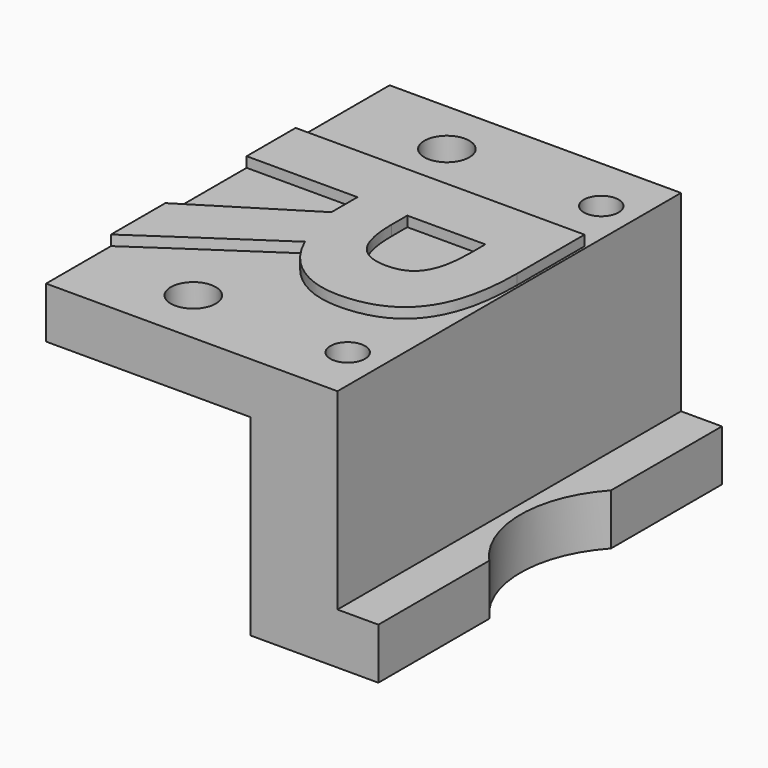
from build123d import *

# Parameters (mm, degrees)
F1_DEPTH     = 42
F2_R         = 1.7
F2_R_2       = 11
F3_DEPTH     = 23.801
F4_W         = 42
F4_H         = 5
F5_DEPTH     = 20
F6_R         = 2.2
F7_DEPTH     = 25
F8_TEXT_SIZE = 39.5833333333
F9_DEPTH     = 1


# Not quite as in the source:
# - Text() gives the source's letters only with a copy of the font that has no kerning and outlines rounded to 1/6400 em; it was checked with that copy


with BuildPart() as f1:
    # F0 (on Front) → F1 (new body)
    with BuildSketch(Plane.XZ):
        Polygon((8.5, 5), (8.5, 23.8), (0, 23.8), (0, 0), (12.5, 0), (12.5, 5), align=None)
    extrude(amount=-F1_DEPTH)

    # F2 (on face) → F3 (cut, through all)
    with BuildSketch(Plane(origin=(0, 0, 0), x_dir=(1, 0, 0), z_dir=(0, 0, -1))):
        with Locations((5.1, -5.5)):
            Circle(F2_R)
        with Locations((5.1, -36.5)):
            Circle(F2_R)
        with Locations((20.6, -21)):
            Circle(F2_R_2)
    extrude(amount=-F3_DEPTH, mode=Mode.SUBTRACT)

    # F4 (on face) → F5 (join)
    with BuildSketch(Plane(origin=(0, 0, 0), x_dir=(0, -1, 0), z_dir=(-1, 0, 0))):
        with Locations((-21, 21.3)):
            Rectangle(F4_W, F4_H)
    extrude(amount=F5_DEPTH)

    # F6 (on face) → F7 (cut)
    with BuildSketch(Plane.XY.offset(23.8)):
        with Locations((-10, 36.5)):
            Circle(F6_R)
        with Locations((-10, 5.5)):
            Circle(F6_R)
    extrude(amount=-F7_DEPTH, mode=Mode.SUBTRACT)

    # F8 (on face) → F9 (join)
    with BuildSketch(Plane.XY.offset(23.8)):
        with Locations(Location((-20, 34.0655924479), (0, 0, -90))):
            Text('R', F8_TEXT_SIZE, font='Open Sans', font_style=FontStyle.BOLD, text_align=(TextAlign.LEFT, TextAlign.BOTTOM))
    extrude(amount=F9_DEPTH)


solid = f1.part
